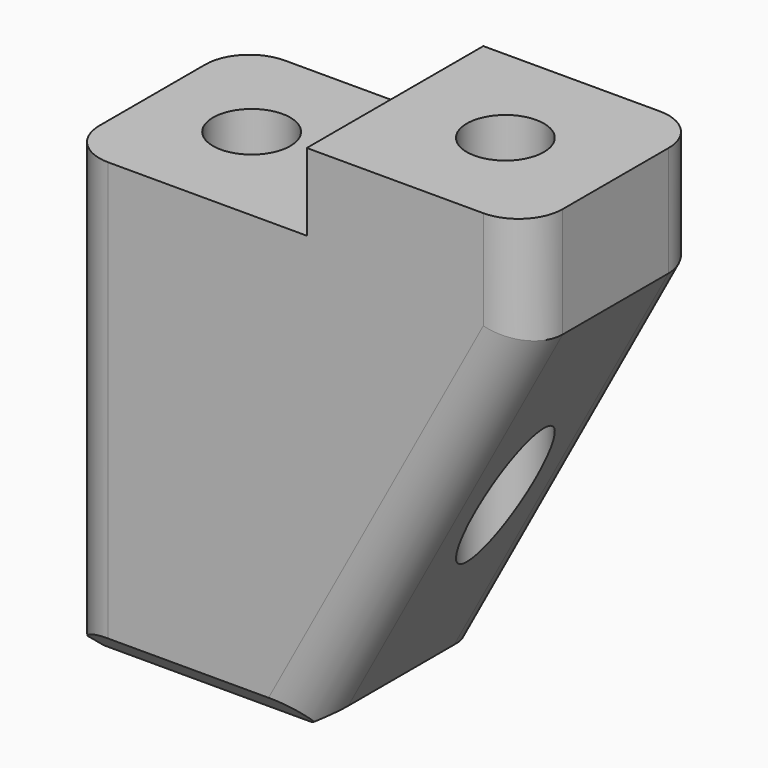
from build123d import *

# Parameters (mm, degrees)
F1_DEPTH    = 5
F2_R        = 1.75
F3_DEPTH    = 23.501
F4_T1_DEPTH = 15.1433659759
F4_T3_DEPTH = 16.1433659759
F4_T5_DEPTH = 13.1544598894
F5_R        = 2


# Not quite as in the source:
# - a fillet or chamfer that OpenCascade refuses, or shapes differently, is made with other operations: its cross-section is extruded or revolved along the edge and cut away or added


with BuildPart() as f1:
    # F0 (on Front) → F1 (new body, symmetric)
    with BuildSketch(Plane.XZ):
        Polygon((0, 3.5), (0, 0), (-11, 0), (-11, -20), (0, -20), (10, -1.5), (10, 3.5), align=None)
    extrude(amount=F1_DEPTH, both=True)

    # F2 (on face) → F3 (cut, through all)
    with BuildSketch(Plane.XY.offset(3.5)):
        with Locations((-6.5, 0)):
            Circle(F2_R)
        with Locations((5, 0)):
            Circle(F2_R)
    extrude(amount=-F3_DEPTH, mode=Mode.SUBTRACT)

    # F4: chamfer of 1 on 5 edges, made by hand

    # F4_s2 → F4_t1 (cut)
    with BuildSketch(Plane.XZ.offset(-7.571682988)):
        Polygon((-11, -19), (-10, -20), (-11, -20), align=None)
    extrude(amount=F4_T1_DEPTH, mode=Mode.SUBTRACT)

    # F4_s4 → F4_t3 (cut)
    with BuildSketch(Plane.YZ.offset(-13.571682988)):
        Polygon((5, -19), (4, -20), (5, -20), align=None)
        Polygon((-5, -19), (-4, -20), (-5, -20), align=None)
    extrude(amount=F4_T3_DEPTH, mode=Mode.SUBTRACT)

    # F4_s6 → F4_t5 (cut)
    with BuildSketch(Plane.XZ.offset(-6.5772299447)):
        Polygon((-0.5962022078, -20), (0.2835043057, -19.4755170344), (0, -20), align=None)
    extrude(amount=F4_T5_DEPTH, mode=Mode.SUBTRACT)

    # F4_s7 → F4_t8 (revolve, cut)
    with BuildSketch(Plane.XZ):
        Polygon((-3.75, -20), (-4.75, -19), (-4.75, -20), align=None)
    revolve(axis=Axis((-6.5, 0, -20), (0, 0, 1)), mode=Mode.SUBTRACT)

    # F5
    f5_edges = [f1.edges().sort_by_distance(p)[0] for p in [
        (-11, -5, -9.5),
        (-11, 5, -9.5),
        (5.27027, -5, -10.25),
        (10, -5, 1),
        (10, 5, 1),
        (5.27027, 5, -10.25),
    ]]
    fillet(f5_edges, radius=F5_R)


solid = f1.part
